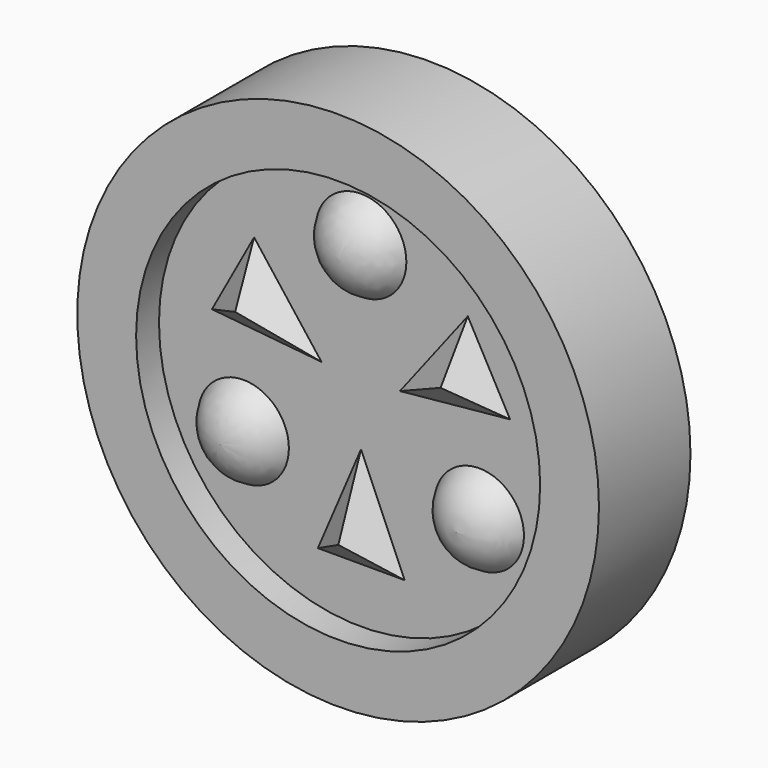
from build123d import *

# Parameters (mm, degrees)
F0_R          = 57.9269385224
F0_R_2        = 45.238930614
F0_R_3        = 10.232456426
F0_R_4        = 9.9260337363
F0_R_5        = 10.3400506536
F1_DEPTH      = 12.7
F2_DEPTH      = 12.7
F3_R          = 44.8601198224
F4_DEPTH      = 6.35
F5_R          = 44.7159015694
F6_DEPTH      = 6.35
F7_R          = 10.0743297083
F7_R_2        = 9.9496681994
F7_R_3        = 10.0826621072
F8_DEPTH      = 6.35
F13_DEPTH     = 6.35
F14_T4_DEPTH  = 74.4109063998
F14_T11_DEPTH = 74.5717160691
F14_T18_DEPTH = 67.9697661213
F14_T26_DEPTH = 74.4109063998
F14_T31_DEPTH = 67.9697661213
F14_T39_DEPTH = 74.4109063998
F14_T44_DEPTH = 74.5717160691
F14_T52_DEPTH = 74.5717160691
F14_T57_DEPTH = 67.9697661213
F15_T4_DEPTH  = 74.5533850225
F15_T11_DEPTH = 67.988668277
F15_T18_DEPTH = 74.6646190403
F15_T26_DEPTH = 74.5533850225
F15_T31_DEPTH = 74.6646190403
F15_T39_DEPTH = 74.5533850225
F15_T44_DEPTH = 67.988668277
F15_T52_DEPTH = 74.6646190403
F15_T57_DEPTH = 67.988668277
F16_T4_DEPTH  = 74.2472188603
F16_T10_DEPTH = 74.1921905859
F16_T16_DEPTH = 67.5143742402
F18_DEPTH     = 6.35
F20_DEPTH     = 6.35


# Not quite as in the source:
# - a fillet or chamfer that OpenCascade refuses, or shapes differently, is made with other operations: its cross-section is extruded or revolved along the edge and cut away or added


with BuildPart() as f1:
    # F0 (on Front) → F1 (new body)
    with BuildSketch(Plane.XZ):
        Circle(F0_R)
        Circle(F0_R_2, mode=Mode.SUBTRACT)
        Circle(F0_R_2)
        with Locations((-26.1295642704, -15.3669575229)):
            Circle(F0_R_3, mode=Mode.SUBTRACT)
        Polygon((-12.544834055, -34.5090515912), (0, -5.3877583705), (12.6424450427, -34.5090515912), align=None, mode=Mode.SUBTRACT)
        with Locations((26.1333119124, -15.1850637048)):
            Circle(F0_R_4, mode=Mode.SUBTRACT)
        Polygon((-36.0336452723, 4.8764180392), (-24.01153557, 26.9035063684), (-4.5260344632, 1.7700339667), align=None, mode=Mode.SUBTRACT)
        Polygon((36.1581519246, 4.842239432), (4.4649434276, 1.758374623), (24.0084677935, 26.875147596), align=None, mode=Mode.SUBTRACT)
        with Locations((0, 29.5979101211)):
            Circle(F0_R_5, mode=Mode.SUBTRACT)
        with Locations((0, 29.5979101211)):
            Circle(F0_R_5)
        Polygon((-4.5260344632, 1.7700339667), (-24.01153557, 26.9035063684), (-36.0336452723, 4.8764180392), align=None)
        with Locations((-26.1295642704, -15.3669575229)):
            Circle(F0_R_3)
        Polygon((12.6424450427, -34.5090515912), (0, -5.3877583705), (-12.544834055, -34.5090515912), align=None)
        with Locations((26.1333119124, -15.1850637048)):
            Circle(F0_R_4)
        Polygon((24.0084677935, 26.875147596), (4.4649434276, 1.758374623), (36.1581519246, 4.842239432), align=None)
    extrude(amount=F1_DEPTH)

    # F2 (add): a face of the model
    f2_faces = [f1.faces().sort_by_distance(p)[0] for p in [
        (0, 0, 0),
    ]]
    extrude(f2_faces, amount=F2_DEPTH)

    # F3 (on face) → F4 (cut)
    with BuildSketch(Plane.XZ.offset(12.7)):
        Circle(F3_R)
    extrude(amount=-F4_DEPTH, mode=Mode.SUBTRACT)

    # F5 (on face) → F6 (cut)
    with BuildSketch(Plane(origin=(0, 12.7, 0), x_dir=(-1, 0, 0), z_dir=(0, 1, 0))):
        Circle(F5_R)
    extrude(amount=-F6_DEPTH, mode=Mode.SUBTRACT)

    # F7 (on face) → F8 (join)
    with BuildSketch(Plane.XZ.offset(6.35)):
        with Locations((0, 29.6977050602)):
            Circle(F7_R)
        with Locations((26.2417513877, -15.2999386191)):
            Circle(F7_R_2)
        with Locations((-26.0976161808, -15.1815246791)):
            Circle(F7_R_3)
    extrude(amount=F8_DEPTH)

    # F9: fillet of radius 11.0998 on 1 edges, made by hand

    # F9_s1 → F9_t2 (revolve, cut)
    with BuildSketch(Plane.XY.offset(29.6977050602)):
        with BuildLine():
            ThreePointArc((10.0743297083, -6.35), (5.9786194513, -10.9790962592), (0.0421335379, -12.7))
            Line((0.0421335379, -12.7), (10.0743297083, -12.7))
            Line((10.0743297083, -12.7), (10.0743297083, -6.35))
        make_face()
    revolve(axis=Axis((0, -12.7, 29.6977050602), (0, -1, 0)), mode=Mode.SUBTRACT)

    # F10: fillet of radius 11.0998 on 1 edges, made by hand

    # F10_s1 → F10_t2 (revolve, cut)
    with BuildSketch(Plane.XY.offset(-15.1815246791)):
        with BuildLine():
            ThreePointArc((-16.0149540736, -6.35), (-20.1106643305, -10.9790962592), (-26.0471502439, -12.7))
            Line((-26.0471502439, -12.7), (-16.0149540736, -12.7))
            Line((-16.0149540736, -12.7), (-16.0149540736, -6.35))
        make_face()
    revolve(axis=Axis((-26.0976161808, -12.7, -15.1815246791), (0, -1, 0)), mode=Mode.SUBTRACT)

    # F11: fillet of radius 10.8204 on 1 edges, made by hand

    # F11_s1 → F11_t2 (revolve, cut)
    with BuildSketch(Plane.XY.offset(-15.2999386191)):
        with BuildLine():
            ThreePointArc((36.1914195871, -6.35), (32.1989541242, -10.9749991754), (26.3376598985, -12.7))
            Line((26.3376598985, -12.7), (36.1914195871, -12.7))
            Line((36.1914195871, -12.7), (36.1914195871, -6.35))
        make_face()
    revolve(axis=Axis((26.2417513877, -12.7, -15.2999386191), (0, -1, 0)), mode=Mode.SUBTRACT)

    # F12 (on face) → F13 (join)
    with BuildSketch(Plane.XZ.offset(6.35)):
        Polygon((-4.5254253782, 1.6911323182), (-24.0121241659, 27.0516239107), (-36.1962728202, 4.7867787071), align=None)
        Polygon((36.2073592842, 4.7867787071), (23.9838846028, 27.0516239107), (4.3973103166, 1.6507724067), align=None)
        Polygon((12.5976987183, -34.5319546759), (0, -5.3459731862), (-12.4581893906, -34.5319546759), align=None)
    extrude(amount=F13_DEPTH)

    # F14: chamfer of 8.2804 on 3 edges, made by hand


with BuildPart() as f14_tool2:
    # F14_s3 → F14_t4 (new body)
    with BuildSketch(Plane(origin=(-57.5107438509, 0, 5.6213502606), x_dir=(0, 1, 0), z_dir=(0.9952569801, 0, -0.0972807463))):
        with BuildLine():
            Line((-4.1853949204, 1.008669406), (-12.9342050796, 9.7574795653))
            Line((-12.9342050796, 9.7574795653), (-13.0998130796, 9.7574795653))
            ThreePointArc((-13.0998130796, 9.7574795653), (-12.865608, 5.5001770255), (-12.865608, 1.2428744857))
            Line((-12.865608, 1.2428744857), (-12.7, 1.0772664857))
            ThreePointArc((-12.7, 1.0772664857), (-8.4426974602, 1.0772664857), (-4.1853949204, 0.843061406))
            Line((-4.1853949204, 0.843061406), (-4.1853949204, 1.008669406))
        make_face()
    extrude(amount=F14_T4_DEPTH)

    split(bisect_by=Plane.XZ.offset(6.35), keep=Keep.TOP)

    split(bisect_by=Plane(origin=(-29.8705033929, 0, 16.3462467576), x_dir=(0, 1, 0), z_dir=(0.8772373953, 0, -0.4800568219)), keep=Keep.TOP)

    split(bisect_by=Plane(origin=(-2.0283818724, 0, -1.5585844001), x_dir=(0, 1, 0), z_dir=(-0.7929468135, 0, -0.6092908591)), keep=Keep.TOP)


with BuildPart() as f1_1:
    add(f1.part)

    # F14_t1: cut F14_tool2
    add(f14_tool2.part, mode=Mode.SUBTRACT)


with BuildPart() as f14_tool9:
    # F14_s10 → F14_t11 (new body)
    with BuildSketch(Plane(origin=(10.477539574, 0, -13.6357398024), x_dir=(0, 1, 0), z_dir=(-0.6092908591, 0, 0.7929468135))):
        with BuildLine():
            Line((-4.1853949204, 2.3238250907), (-12.9342050796, 11.07263525))
            Line((-12.9342050796, 11.07263525), (-13.0998130796, 11.07263525))
            ThreePointArc((-13.0998130796, 11.07263525), (-12.865608, 6.8153327102), (-12.865608, 2.5580301704))
            Line((-12.865608, 2.5580301704), (-12.7, 2.3924221704))
            ThreePointArc((-12.7, 2.3924221704), (-8.4426974602, 2.3924221704), (-4.1853949204, 2.1582170907))
            Line((-4.1853949204, 2.1582170907), (-4.1853949204, 2.3238250907))
        make_face()
    extrude(amount=F14_T11_DEPTH)

    split(bisect_by=Plane.XZ.offset(6.35), keep=Keep.TOP)

    split(bisect_by=Plane(origin=(0.1209077576, 0, 1.2369795072), x_dir=(0, 1, 0), z_dir=(0.0972807463, 0, 0.9952569801)), keep=Keep.TOP)

    split(bisect_by=Plane(origin=(-29.8705033929, 0, 16.3462467576), x_dir=(0, 1, 0), z_dir=(0.8772373953, 0, -0.4800568219)), keep=Keep.TOP)


with BuildPart() as f1_2:
    add(f1_1.part)

    # F14_t8: cut F14_tool9
    add(f14_tool9.part, mode=Mode.SUBTRACT)


with BuildPart() as f14_tool16:
    # F14_s17 → F14_t18 (new body)
    with BuildSketch(Plane(origin=(16.080979856, 0, 29.3857648468), x_dir=(0, 1, 0), z_dir=(-0.4800568219, 0, -0.8772373953))):
        with BuildLine():
            Line((-4.1853949204, -34.2848549414), (-12.9342050796, -25.5360447821))
            Line((-12.9342050796, -25.5360447821), (-13.0998130796, -25.5360447821))
            ThreePointArc((-13.0998130796, -25.5360447821), (-12.865608, -29.7933473219), (-12.865608, -34.0506498617))
            Line((-12.865608, -34.0506498617), (-12.7, -34.2162578617))
            ThreePointArc((-12.7, -34.2162578617), (-8.4426974602, -34.2162578617), (-4.1853949204, -34.4504629414))
            Line((-4.1853949204, -34.4504629414), (-4.1853949204, -34.2848549414))
        make_face()
    extrude(amount=F14_T18_DEPTH)

    split(bisect_by=Plane.XZ.offset(6.35), keep=Keep.TOP)

    split(bisect_by=Plane(origin=(0.1209077576, 0, 1.2369795072), x_dir=(0, 1, 0), z_dir=(0.0972807463, 0, 0.9952569801)), keep=Keep.TOP)

    split(bisect_by=Plane(origin=(-2.0283818724, 0, -1.5585844001), x_dir=(0, 1, 0), z_dir=(-0.7929468135, 0, -0.6092908591)), keep=Keep.TOP)


with BuildPart() as f1_3:
    add(f1_2.part)

    # F14_t15: cut F14_tool16
    add(f14_tool16.part, mode=Mode.SUBTRACT)


with BuildPart() as f14_tool24:
    # F14_s25 → F14_t26 (new body)
    with BuildSketch(Plane(origin=(-57.5107438509, 0, 5.6213502606), x_dir=(0, 1, 0), z_dir=(0.9952569801, 0, -0.0972807463))):
        with BuildLine():
            Line((-4.1853949204, 1.008669406), (-12.9342050796, 9.7574795653))
            Line((-12.9342050796, 9.7574795653), (-13.0998130796, 9.7574795653))
            ThreePointArc((-13.0998130796, 9.7574795653), (-12.865608, 5.5001770255), (-12.865608, 1.2428744857))
            Line((-12.865608, 1.2428744857), (-12.7, 1.0772664857))
            ThreePointArc((-12.7, 1.0772664857), (-8.4426974602, 1.0772664857), (-4.1853949204, 0.843061406))
            Line((-4.1853949204, 0.843061406), (-4.1853949204, 1.008669406))
        make_face()
    extrude(amount=F14_T26_DEPTH)

    split(bisect_by=Plane.XZ.offset(6.35), keep=Keep.TOP)

    split(bisect_by=Plane(origin=(-29.8705033929, 0, 16.3462467576), x_dir=(0, 1, 0), z_dir=(-0.8772373953, 0, 0.4800568219)), keep=Keep.TOP)


with BuildPart() as f14_tool29:
    # F14_s30 → F14_t31 (new body)
    with BuildSketch(Plane(origin=(16.080979856, 0, 29.3857648468), x_dir=(0, 1, 0), z_dir=(-0.4800568219, 0, -0.8772373953))):
        with BuildLine():
            Line((-4.1853949204, -34.2848549414), (-12.9342050796, -25.5360447821))
            Line((-12.9342050796, -25.5360447821), (-13.0998130796, -25.5360447821))
            ThreePointArc((-13.0998130796, -25.5360447821), (-12.865608, -29.7933473219), (-12.865608, -34.0506498617))
            Line((-12.865608, -34.0506498617), (-12.7, -34.2162578617))
            ThreePointArc((-12.7, -34.2162578617), (-8.4426974602, -34.2162578617), (-4.1853949204, -34.4504629414))
            Line((-4.1853949204, -34.4504629414), (-4.1853949204, -34.2848549414))
        make_face()
    extrude(amount=F14_T31_DEPTH)

    split(bisect_by=Plane.XZ.offset(6.35), keep=Keep.TOP)

    split(bisect_by=Plane(origin=(0.1209077576, 0, 1.2369795072), x_dir=(0, 1, 0), z_dir=(-0.0972807463, 0, -0.9952569801)), keep=Keep.TOP)


with BuildPart() as f14_tool24_1:
    add(f14_tool24.part)

    # F14_t34: intersect F14_tool29
    add(f14_tool29.part, mode=Mode.INTERSECT)


with BuildPart() as f1_4:
    add(f1_3.part)

    # F14_t22: cut F14_tool24
    add(f14_tool24_1.part, mode=Mode.SUBTRACT)


with BuildPart() as f14_tool37:
    # F14_s38 → F14_t39 (new body)
    with BuildSketch(Plane(origin=(-57.5107438509, 0, 5.6213502606), x_dir=(0, 1, 0), z_dir=(0.9952569801, 0, -0.0972807463))):
        with BuildLine():
            Line((-4.1853949204, 1.008669406), (-12.9342050796, 9.7574795653))
            Line((-12.9342050796, 9.7574795653), (-13.0998130796, 9.7574795653))
            ThreePointArc((-13.0998130796, 9.7574795653), (-12.865608, 5.5001770255), (-12.865608, 1.2428744857))
            Line((-12.865608, 1.2428744857), (-12.7, 1.0772664857))
            ThreePointArc((-12.7, 1.0772664857), (-8.4426974602, 1.0772664857), (-4.1853949204, 0.843061406))
            Line((-4.1853949204, 0.843061406), (-4.1853949204, 1.008669406))
        make_face()
    extrude(amount=F14_T39_DEPTH)

    split(bisect_by=Plane.XZ.offset(6.35), keep=Keep.TOP)

    split(bisect_by=Plane(origin=(-2.0283818724, 0, -1.5585844001), x_dir=(0, 1, 0), z_dir=(0.7929468135, 0, 0.6092908591)), keep=Keep.TOP)


with BuildPart() as f14_tool42:
    # F14_s43 → F14_t44 (new body)
    with BuildSketch(Plane(origin=(10.477539574, 0, -13.6357398024), x_dir=(0, 1, 0), z_dir=(-0.6092908591, 0, 0.7929468135))):
        with BuildLine():
            Line((-4.1853949204, 2.3238250907), (-12.9342050796, 11.07263525))
            Line((-12.9342050796, 11.07263525), (-13.0998130796, 11.07263525))
            ThreePointArc((-13.0998130796, 11.07263525), (-12.865608, 6.8153327102), (-12.865608, 2.5580301704))
            Line((-12.865608, 2.5580301704), (-12.7, 2.3924221704))
            ThreePointArc((-12.7, 2.3924221704), (-8.4426974602, 2.3924221704), (-4.1853949204, 2.1582170907))
            Line((-4.1853949204, 2.1582170907), (-4.1853949204, 2.3238250907))
        make_face()
    extrude(amount=F14_T44_DEPTH)

    split(bisect_by=Plane.XZ.offset(6.35), keep=Keep.TOP)

    split(bisect_by=Plane(origin=(0.1209077576, 0, 1.2369795072), x_dir=(0, 1, 0), z_dir=(-0.0972807463, 0, -0.9952569801)), keep=Keep.TOP)


with BuildPart() as f14_tool37_1:
    add(f14_tool37.part)

    # F14_t47: intersect F14_tool42
    add(f14_tool42.part, mode=Mode.INTERSECT)


with BuildPart() as f1_5:
    add(f1_4.part)

    # F14_t35: cut F14_tool37
    add(f14_tool37_1.part, mode=Mode.SUBTRACT)


with BuildPart() as f14_tool50:
    # F14_s51 → F14_t52 (new body)
    with BuildSketch(Plane(origin=(10.477539574, 0, -13.6357398024), x_dir=(0, 1, 0), z_dir=(-0.6092908591, 0, 0.7929468135))):
        with BuildLine():
            Line((-4.1853949204, 2.3238250907), (-12.9342050796, 11.07263525))
            Line((-12.9342050796, 11.07263525), (-13.0998130796, 11.07263525))
            ThreePointArc((-13.0998130796, 11.07263525), (-12.865608, 6.8153327102), (-12.865608, 2.5580301704))
            Line((-12.865608, 2.5580301704), (-12.7, 2.3924221704))
            ThreePointArc((-12.7, 2.3924221704), (-8.4426974602, 2.3924221704), (-4.1853949204, 2.1582170907))
            Line((-4.1853949204, 2.1582170907), (-4.1853949204, 2.3238250907))
        make_face()
    extrude(amount=F14_T52_DEPTH)

    split(bisect_by=Plane.XZ.offset(6.35), keep=Keep.TOP)

    split(bisect_by=Plane(origin=(-29.8705033929, 0, 16.3462467576), x_dir=(0, 1, 0), z_dir=(-0.8772373953, 0, 0.4800568219)), keep=Keep.TOP)


with BuildPart() as f14_tool55:
    # F14_s56 → F14_t57 (new body)
    with BuildSketch(Plane(origin=(16.080979856, 0, 29.3857648468), x_dir=(0, 1, 0), z_dir=(-0.4800568219, 0, -0.8772373953))):
        with BuildLine():
            Line((-4.1853949204, -34.2848549414), (-12.9342050796, -25.5360447821))
            Line((-12.9342050796, -25.5360447821), (-13.0998130796, -25.5360447821))
            ThreePointArc((-13.0998130796, -25.5360447821), (-12.865608, -29.7933473219), (-12.865608, -34.0506498617))
            Line((-12.865608, -34.0506498617), (-12.7, -34.2162578617))
            ThreePointArc((-12.7, -34.2162578617), (-8.4426974602, -34.2162578617), (-4.1853949204, -34.4504629414))
            Line((-4.1853949204, -34.4504629414), (-4.1853949204, -34.2848549414))
        make_face()
    extrude(amount=F14_T57_DEPTH)

    split(bisect_by=Plane.XZ.offset(6.35), keep=Keep.TOP)

    split(bisect_by=Plane(origin=(-2.0283818724, 0, -1.5585844001), x_dir=(0, 1, 0), z_dir=(0.7929468135, 0, 0.6092908591)), keep=Keep.TOP)


with BuildPart() as f14_tool50_1:
    add(f14_tool50.part)

    # F14_t60: intersect F14_tool55
    add(f14_tool55.part, mode=Mode.INTERSECT)


with BuildPart() as f1_6:
    add(f1_5.part)

    # F14_t48: cut F14_tool50
    add(f14_tool50_1.part, mode=Mode.SUBTRACT)

    # F15: chamfer of 8.2804 on 3 edges, made by hand


with BuildPart() as f15_tool2:
    # F15_s3 → F15_t4 (new body)
    with BuildSketch(Plane(origin=(-16.6756708248, 0, -1.6439776255), x_dir=(0, 1, 0), z_dir=(0.995175598, 0, 0.0981097812))):
        with BuildLine():
            Line((-4.1853949204, 0.9771841842), (-12.9342050796, 9.7259943435))
            Line((-12.9342050796, 9.7259943435), (-13.0998130796, 9.7259943435))
            ThreePointArc((-13.0998130796, 9.7259943435), (-12.865608, 5.4686918036), (-12.865608, 1.2113892638))
            Line((-12.865608, 1.2113892638), (-12.7, 1.0457812638))
            ThreePointArc((-12.7, 1.0457812638), (-8.4426974602, 1.0457812638), (-4.1853949204, 0.8115761842))
            Line((-4.1853949204, 0.8115761842), (-4.1853949204, 0.9771841842))
        make_face()
    extrude(amount=F15_T4_DEPTH)

    split(bisect_by=Plane.XZ.offset(6.35), keep=Keep.TOP)

    split(bisect_by=Plane(origin=(1.9593711293, 0, -1.510869357), x_dir=(0, 1, 0), z_dir=(0.7919084131, 0, -0.6106398818)), keep=Keep.TOP)

    split(bisect_by=Plane(origin=(29.8410766305, 0, 16.3828511415), x_dir=(0, 1, 0), z_dir=(-0.8765845615, 0, -0.4812478639)), keep=Keep.TOP)


with BuildPart() as f1_7:
    add(f1_6.part)

    # F15_t1: cut F15_tool2
    add(f15_tool2.part, mode=Mode.SUBTRACT)


with BuildPart() as f15_tool9:
    # F15_s10 → F15_t11 (new body)
    with BuildSketch(Plane(origin=(16.6142460012, 0, -30.2625583178), x_dir=(0, 1, 0), z_dir=(-0.4812478639, 0, 0.8765845615))):
        with BuildLine():
            Line((-4.1853949204, -34.2766442695), (-12.9342050796, -25.5278341102))
            Line((-12.9342050796, -25.5278341102), (-13.0998130796, -25.5278341102))
            ThreePointArc((-13.0998130796, -25.5278341102), (-12.865608, -29.78513665), (-12.865608, -34.0424391898))
            Line((-12.865608, -34.0424391898), (-12.7, -34.2080471898))
            ThreePointArc((-12.7, -34.2080471898), (-8.4426974602, -34.2080471898), (-4.1853949204, -34.4422522695))
            Line((-4.1853949204, -34.4422522695), (-4.1853949204, -34.2766442695))
        make_face()
    extrude(amount=F15_T11_DEPTH)

    split(bisect_by=Plane.XZ.offset(6.35), keep=Keep.TOP)

    split(bisect_by=Plane(origin=(-0.1188491357, 0, 1.205545035), x_dir=(0, 1, 0), z_dir=(-0.0981097812, 0, 0.995175598)), keep=Keep.TOP)

    split(bisect_by=Plane(origin=(1.9593711293, 0, -1.510869357), x_dir=(0, 1, 0), z_dir=(0.7919084131, 0, -0.6106398818)), keep=Keep.TOP)


with BuildPart() as f1_8:
    add(f1_7.part)

    # F15_t8: cut F15_tool9
    add(f15_tool9.part, mode=Mode.SUBTRACT)


with BuildPart() as f15_tool16:
    # F15_s17 → F15_t18 (new body)
    with BuildSketch(Plane(origin=(35.0278234042, 0, 45.4258375046), x_dir=(0, 1, 0), z_dir=(-0.6106398818, 0, -0.7919084131))):
        with BuildLine():
            Line((-4.1853949204, 2.2400344876), (-12.9342050796, 10.9888446469))
            Line((-12.9342050796, 10.9888446469), (-13.0998130796, 10.9888446469))
            ThreePointArc((-13.0998130796, 10.9888446469), (-12.865608, 6.7315421071), (-12.865608, 2.4742395673))
            Line((-12.865608, 2.4742395673), (-12.7, 2.3086315673))
            ThreePointArc((-12.7, 2.3086315673), (-8.4426974602, 2.3086315673), (-4.1853949204, 2.0744264876))
            Line((-4.1853949204, 2.0744264876), (-4.1853949204, 2.2400344876))
        make_face()
    extrude(amount=F15_T18_DEPTH)

    split(bisect_by=Plane.XZ.offset(6.35), keep=Keep.TOP)

    split(bisect_by=Plane(origin=(-0.1188491357, 0, 1.205545035), x_dir=(0, 1, 0), z_dir=(-0.0981097812, 0, 0.995175598)), keep=Keep.TOP)

    split(bisect_by=Plane(origin=(29.8410766305, 0, 16.3828511415), x_dir=(0, 1, 0), z_dir=(-0.8765845615, 0, -0.4812478639)), keep=Keep.TOP)


with BuildPart() as f1_9:
    add(f1_8.part)

    # F15_t15: cut F15_tool16
    add(f15_tool16.part, mode=Mode.SUBTRACT)


with BuildPart() as f15_tool24:
    # F15_s25 → F15_t26 (new body)
    with BuildSketch(Plane(origin=(-16.6756708248, 0, -1.6439776255), x_dir=(0, 1, 0), z_dir=(0.995175598, 0, 0.0981097812))):
        with BuildLine():
            Line((-4.1853949204, 0.9771841842), (-12.9342050796, 9.7259943435))
            Line((-12.9342050796, 9.7259943435), (-13.0998130796, 9.7259943435))
            ThreePointArc((-13.0998130796, 9.7259943435), (-12.865608, 5.4686918036), (-12.865608, 1.2113892638))
            Line((-12.865608, 1.2113892638), (-12.7, 1.0457812638))
            ThreePointArc((-12.7, 1.0457812638), (-8.4426974602, 1.0457812638), (-4.1853949204, 0.8115761842))
            Line((-4.1853949204, 0.8115761842), (-4.1853949204, 0.9771841842))
        make_face()
    extrude(amount=F15_T26_DEPTH)

    split(bisect_by=Plane.XZ.offset(6.35), keep=Keep.TOP)

    split(bisect_by=Plane(origin=(1.9593711293, 0, -1.510869357), x_dir=(0, 1, 0), z_dir=(-0.7919084131, 0, 0.6106398818)), keep=Keep.TOP)


with BuildPart() as f15_tool29:
    # F15_s30 → F15_t31 (new body)
    with BuildSketch(Plane(origin=(35.0278234042, 0, 45.4258375046), x_dir=(0, 1, 0), z_dir=(-0.6106398818, 0, -0.7919084131))):
        with BuildLine():
            Line((-4.1853949204, 2.2400344876), (-12.9342050796, 10.9888446469))
            Line((-12.9342050796, 10.9888446469), (-13.0998130796, 10.9888446469))
            ThreePointArc((-13.0998130796, 10.9888446469), (-12.865608, 6.7315421071), (-12.865608, 2.4742395673))
            Line((-12.865608, 2.4742395673), (-12.7, 2.3086315673))
            ThreePointArc((-12.7, 2.3086315673), (-8.4426974602, 2.3086315673), (-4.1853949204, 2.0744264876))
            Line((-4.1853949204, 2.0744264876), (-4.1853949204, 2.2400344876))
        make_face()
    extrude(amount=F15_T31_DEPTH)

    split(bisect_by=Plane.XZ.offset(6.35), keep=Keep.TOP)

    split(bisect_by=Plane(origin=(-0.1188491357, 0, 1.205545035), x_dir=(0, 1, 0), z_dir=(0.0981097812, 0, -0.995175598)), keep=Keep.TOP)


with BuildPart() as f15_tool24_1:
    add(f15_tool24.part)

    # F15_t34: intersect F15_tool29
    add(f15_tool29.part, mode=Mode.INTERSECT)


with BuildPart() as f1_10:
    add(f1_9.part)

    # F15_t22: cut F15_tool24
    add(f15_tool24_1.part, mode=Mode.SUBTRACT)


with BuildPart() as f15_tool37:
    # F15_s38 → F15_t39 (new body)
    with BuildSketch(Plane(origin=(-16.6756708248, 0, -1.6439776255), x_dir=(0, 1, 0), z_dir=(0.995175598, 0, 0.0981097812))):
        with BuildLine():
            Line((-4.1853949204, 0.9771841842), (-12.9342050796, 9.7259943435))
            Line((-12.9342050796, 9.7259943435), (-13.0998130796, 9.7259943435))
            ThreePointArc((-13.0998130796, 9.7259943435), (-12.865608, 5.4686918036), (-12.865608, 1.2113892638))
            Line((-12.865608, 1.2113892638), (-12.7, 1.0457812638))
            ThreePointArc((-12.7, 1.0457812638), (-8.4426974602, 1.0457812638), (-4.1853949204, 0.8115761842))
            Line((-4.1853949204, 0.8115761842), (-4.1853949204, 0.9771841842))
        make_face()
    extrude(amount=F15_T39_DEPTH)

    split(bisect_by=Plane.XZ.offset(6.35), keep=Keep.TOP)

    split(bisect_by=Plane(origin=(29.8410766305, 0, 16.3828511415), x_dir=(0, 1, 0), z_dir=(0.8765845615, 0, 0.4812478639)), keep=Keep.TOP)


with BuildPart() as f15_tool42:
    # F15_s43 → F15_t44 (new body)
    with BuildSketch(Plane(origin=(16.6142460012, 0, -30.2625583178), x_dir=(0, 1, 0), z_dir=(-0.4812478639, 0, 0.8765845615))):
        with BuildLine():
            Line((-4.1853949204, -34.2766442695), (-12.9342050796, -25.5278341102))
            Line((-12.9342050796, -25.5278341102), (-13.0998130796, -25.5278341102))
            ThreePointArc((-13.0998130796, -25.5278341102), (-12.865608, -29.78513665), (-12.865608, -34.0424391898))
            Line((-12.865608, -34.0424391898), (-12.7, -34.2080471898))
            ThreePointArc((-12.7, -34.2080471898), (-8.4426974602, -34.2080471898), (-4.1853949204, -34.4422522695))
            Line((-4.1853949204, -34.4422522695), (-4.1853949204, -34.2766442695))
        make_face()
    extrude(amount=F15_T44_DEPTH)

    split(bisect_by=Plane.XZ.offset(6.35), keep=Keep.TOP)

    split(bisect_by=Plane(origin=(-0.1188491357, 0, 1.205545035), x_dir=(0, 1, 0), z_dir=(0.0981097812, 0, -0.995175598)), keep=Keep.TOP)


with BuildPart() as f15_tool37_1:
    add(f15_tool37.part)

    # F15_t47: intersect F15_tool42
    add(f15_tool42.part, mode=Mode.INTERSECT)


with BuildPart() as f1_11:
    add(f1_10.part)

    # F15_t35: cut F15_tool37
    add(f15_tool37_1.part, mode=Mode.SUBTRACT)


with BuildPart() as f15_tool50:
    # F15_s51 → F15_t52 (new body)
    with BuildSketch(Plane(origin=(35.0278234042, 0, 45.4258375046), x_dir=(0, 1, 0), z_dir=(-0.6106398818, 0, -0.7919084131))):
        with BuildLine():
            Line((-4.1853949204, 2.2400344876), (-12.9342050796, 10.9888446469))
            Line((-12.9342050796, 10.9888446469), (-13.0998130796, 10.9888446469))
            ThreePointArc((-13.0998130796, 10.9888446469), (-12.865608, 6.7315421071), (-12.865608, 2.4742395673))
            Line((-12.865608, 2.4742395673), (-12.7, 2.3086315673))
            ThreePointArc((-12.7, 2.3086315673), (-8.4426974602, 2.3086315673), (-4.1853949204, 2.0744264876))
            Line((-4.1853949204, 2.0744264876), (-4.1853949204, 2.2400344876))
        make_face()
    extrude(amount=F15_T52_DEPTH)

    split(bisect_by=Plane.XZ.offset(6.35), keep=Keep.TOP)

    split(bisect_by=Plane(origin=(29.8410766305, 0, 16.3828511415), x_dir=(0, 1, 0), z_dir=(0.8765845615, 0, 0.4812478639)), keep=Keep.TOP)


with BuildPart() as f15_tool55:
    # F15_s56 → F15_t57 (new body)
    with BuildSketch(Plane(origin=(16.6142460012, 0, -30.2625583178), x_dir=(0, 1, 0), z_dir=(-0.4812478639, 0, 0.8765845615))):
        with BuildLine():
            Line((-4.1853949204, -34.2766442695), (-12.9342050796, -25.5278341102))
            Line((-12.9342050796, -25.5278341102), (-13.0998130796, -25.5278341102))
            ThreePointArc((-13.0998130796, -25.5278341102), (-12.865608, -29.78513665), (-12.865608, -34.0424391898))
            Line((-12.865608, -34.0424391898), (-12.7, -34.2080471898))
            ThreePointArc((-12.7, -34.2080471898), (-8.4426974602, -34.2080471898), (-4.1853949204, -34.4422522695))
            Line((-4.1853949204, -34.4422522695), (-4.1853949204, -34.2766442695))
        make_face()
    extrude(amount=F15_T57_DEPTH)

    split(bisect_by=Plane.XZ.offset(6.35), keep=Keep.TOP)

    split(bisect_by=Plane(origin=(1.9593711293, 0, -1.510869357), x_dir=(0, 1, 0), z_dir=(-0.7919084131, 0, 0.6106398818)), keep=Keep.TOP)


with BuildPart() as f15_tool50_1:
    add(f15_tool50.part)

    # F15_t60: intersect F15_tool55
    add(f15_tool55.part, mode=Mode.INTERSECT)


with BuildPart() as f1_12:
    add(f1_11.part)

    # F15_t48: cut F15_tool50
    add(f15_tool50_1.part, mode=Mode.SUBTRACT)

    # F16: chamfer of 8.255 on 3 edges, made by hand


with BuildPart() as f16_tool2:
    # F16_s3 → F16_t4 (new body)
    with BuildSketch(Plane(origin=(22.9558477812, 0, -53.1834395633), x_dir=(0, 1, 0), z_dir=(-0.3962944615, 0, 0.9181234665))):
        Polygon((-4.445, 2.118579565), (-12.7, 10.373579565), (-12.7, 2.118579565), align=None)
    extrude(amount=F16_T4_DEPTH)

    split(bisect_by=Plane.XZ.offset(6.35), keep=Keep.TOP)

    split(bisect_by=Plane.XY.offset(-34.5319546759), keep=Keep.TOP)


with BuildPart() as f1_13:
    add(f1_12.part)

    # F16_t1: cut F16_tool2
    add(f16_tool2.part, mode=Mode.SUBTRACT)


with BuildPart() as f16_tool8:
    # F16_s9 → F16_t10 (new body)
    with BuildSketch(Plane(origin=(6.4040370991, 0, 15.0028308588), x_dir=(0, 1, 0), z_dir=(-0.3925854105, 0, -0.9197155514))):
        Polygon((-4.445, 2.0987510779), (-12.7, 10.3537510779), (-12.7, 2.0987510779), align=None)
    extrude(amount=F16_T10_DEPTH)

    split(bisect_by=Plane.XZ.offset(6.35), keep=Keep.TOP)

    split(bisect_by=Plane.XY.offset(-34.5319546759), keep=Keep.TOP)


with BuildPart() as f1_14:
    add(f1_13.part)

    # F16_t7: cut F16_tool8
    add(f16_tool8.part, mode=Mode.SUBTRACT)


with BuildPart() as f16_tool14:
    # F16_s15 → F16_t16 (new body)
    with BuildSketch(Plane.YZ.offset(-33.6874324563)):
        Polygon((-4.445, -34.5319546759), (-12.7, -26.2769546759), (-12.7, -34.5319546759), align=None)
    extrude(amount=F16_T16_DEPTH)

    split(bisect_by=Plane.XZ.offset(6.35), keep=Keep.TOP)

    split(bisect_by=Plane(origin=(-1.9451176143, 0, -0.8395813478), x_dir=(0, 1, 0), z_dir=(-0.9181234665, 0, -0.3962944615)), keep=Keep.TOP)

    split(bisect_by=Plane(origin=(1.9302540048, 0, -0.8239390535), x_dir=(0, 1, 0), z_dir=(0.9197155514, 0, -0.3925854105)), keep=Keep.TOP)


with BuildPart() as f1_15:
    add(f1_14.part)

    # F16_t13: cut F16_tool14
    add(f16_tool14.part, mode=Mode.SUBTRACT)

    # F17 (on face) → F18 (join)
    with BuildSketch(Plane(origin=(0, 6.35, 0), x_dir=(-1, 0, 0), z_dir=(0, 1, 0))):
        Polygon((0.1139463857, -15.4419038445), (-13.0555815995, 7.0367623121), (-26.1111631989, -15.4419038445), align=None)
        Polygon((0.1139463857, -15.4419038445), (13.1695279852, 7.0367623121), (-13.0555815995, 7.0367623121), align=None)
        Polygon((13.1695279852, 7.0367623121), (0, 29.5154284686), (-13.0555815995, 7.0367623121), align=None)
        Polygon((26.3390559703, -15.4419038445), (13.1695279852, 7.0367623121), (0.1139463857, -15.4419038445), align=None)
    extrude(amount=F18_DEPTH)

    # F19 (on face) → F20 (cut)
    with BuildSketch(Plane(origin=(0, 12.7, 0), x_dir=(-1, 0, 0), z_dir=(0, 1, 0))):
        Polygon((12.9840383306, 6.3451784663), (-12.7162076533, 6.3451784663), (0, -15.0037035346), align=None)
    extrude(amount=-F20_DEPTH, mode=Mode.SUBTRACT)


solid = f1_15.part
